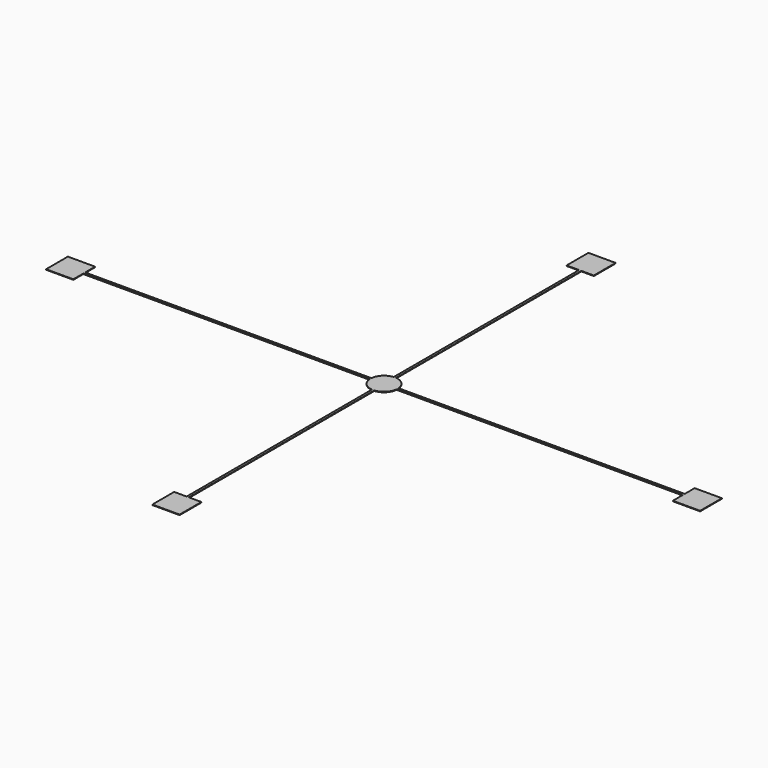
from build123d import *

# Parameters (mm, degrees)
F1_DEPTH = 0.2


# Not quite as in the source:
# - a feature names something its author has since deleted; it is built from what else it names


with BuildPart() as f1:
    # F0 (on Top) → F1 (new body)
    with BuildSketch(Plane.XY):
        Polygon((-110, -0.43), (-110, 0.43), (-110, 5), (-120, 5), (-120, -5), (-110, -5), align=None)
        with BuildLine():
            ThreePointArc((-4.981475685, -0.43), (-5, 0), (-4.981475685, 0.43))
            Line((-4.981475685, 0.43), (-110, 0.43))
            Line((-110, 0.43), (-110, -0.43))
            Line((-110, -0.43), (-4.981475685, -0.43))
        make_face()
        with BuildLine():
            ThreePointArc((-0.43, 4.981475685), (0, 5), (0.43, 4.981475685))
            Line((0.43, 4.981475685), (0.43, 90))
            Line((0.43, 90), (-0.43, 90))
            Line((-0.43, 90), (-0.43, 4.981475685))
        make_face()
        with BuildLine():
            ThreePointArc((4.981475685, 0.43), (4.9953667746, 0.2151994135), (5, 0))
            ThreePointArc((5, 0), (4.9953667746, -0.2151994135), (4.981475685, -0.43))
            Line((4.981475685, -0.43), (110, -0.43))
            Line((110, -0.43), (110, 0.43))
            Line((110, 0.43), (4.981475685, 0.43))
        make_face()
        with BuildLine():
            Line((0.43, -90), (0.43, -4.981475685))
            ThreePointArc((0.43, -4.981475685), (0, -5), (-0.43, -4.981475685))
            Line((-0.43, -4.981475685), (-0.43, -90))
            Line((-0.43, -90), (0.43, -90))
        make_face()
        Polygon((110, 5), (110, 0.43), (110, -0.43), (110, -5), (120, -5), (120, 5), align=None)
        Polygon((5, -90), (0.43, -90), (-0.43, -90), (-5, -90), (-5, -100), (5, -100), align=None)
        Polygon((-0.43, 90), (0.43, 90), (5, 90), (5, 100), (-5, 100), (-5, 90), align=None)
        with BuildLine():
            ThreePointArc((4.981475685, -0.43), (4.9953667746, -0.2151994135), (5, 0))
            ThreePointArc((5, 0), (4.9953667746, 0.2151994135), (4.981475685, 0.43))
            ThreePointArc((4.981475685, 0.43), (3.5355339059, 3.5355339059), (0.43, 4.981475685))
            ThreePointArc((0.43, 4.981475685), (0, 5), (-0.43, 4.981475685))
            ThreePointArc((-0.43, 4.981475685), (-3.5355339059, 3.5355339059), (-4.981475685, 0.43))
            ThreePointArc((-4.981475685, 0.43), (-5, 0), (-4.981475685, -0.43))
            ThreePointArc((-4.981475685, -0.43), (-3.5355339059, -3.5355339059), (-0.43, -4.981475685))
            ThreePointArc((-0.43, -4.981475685), (0, -5), (0.43, -4.981475685))
            ThreePointArc((0.43, -4.981475685), (3.5355339059, -3.5355339059), (4.981475685, -0.43))
        make_face()
    extrude(amount=F1_DEPTH)


solid = f1.part
